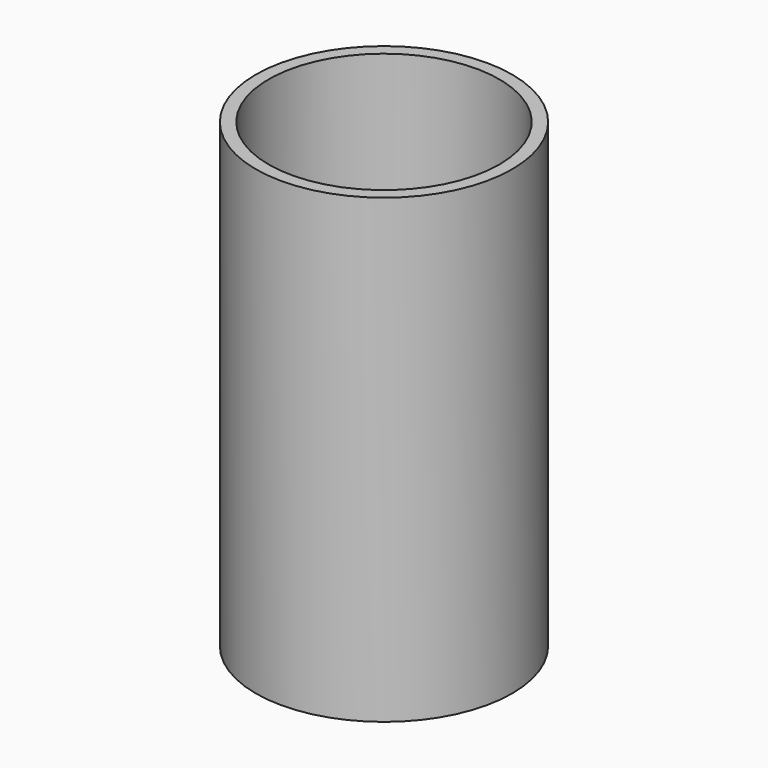
from build123d import *

# Parameters (mm, degrees)
F0_R     = 12.7
F0_R_2   = 11.43
F1_DEPTH = 43.18
F2_R     = 12.7
F2_R_2   = 11.43
F2_R_3   = 1.27
F3_DEPTH = 2.54


with BuildPart() as f1:
    # F0 (on Top) → F1 (new body)
    with BuildSketch(Plane.XY):
        Circle(F0_R)
        Circle(F0_R_2, mode=Mode.SUBTRACT)
    extrude(amount=F1_DEPTH)

    # F2 (on face) → F3 (join)
    with BuildSketch(Plane(origin=(0, 0, 0), x_dir=(1, 0, 0), z_dir=(0, 0, -1))):
        Circle(F2_R)
        Circle(F2_R_2, mode=Mode.SUBTRACT)
        Circle(F2_R_2)
        Circle(F2_R_3, mode=Mode.SUBTRACT)
    extrude(amount=F3_DEPTH)


solid = f1.part
